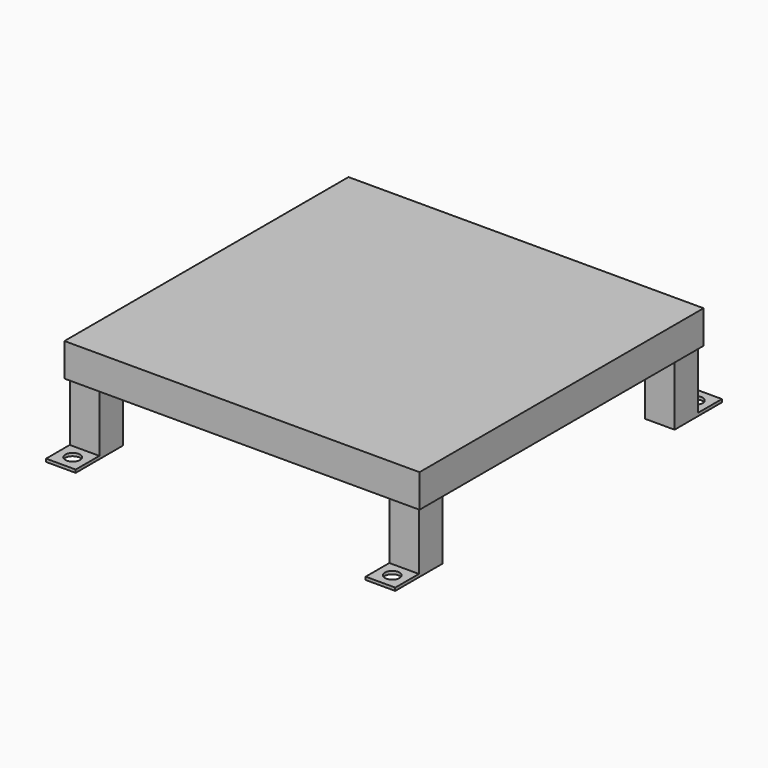
from build123d import *

# Parameters (mm, degrees)
F0_W         = 304.8
F0_H         = 304.8
F1_DEPTH     = 3
F2_W         = 304.8
F2_H         = 304.8
F3_DEPTH     = 25.4
F4_T         = -2.54
F5_W         = 25.4
F5_H         = 25.4
F6_DEPTH     = 76.2
F7_T         = 2.54
F7_T3_DEPTH  = 30.48
F7_T5_DEPTH  = 30.48
F7_T7_DEPTH  = 30.94
F7_T9_DEPTH  = 304.8
F7_T11_DEPTH = 279.4
F7_T13_DEPTH = 279.4
F7_T15_DEPTH = 304.8
F8_W         = 25.4
F8_H         = 25.4
F8_W_2       = 20.32
F8_H_2       = 20.32
F9_DEPTH     = 76.2
F10_W        = 25.4
F10_H        = 50.8
F10_R        = 6.3459053742
F11_DEPTH    = 2.54
F12_W        = 25.4
F12_H        = 50.8
F12_R        = 6.35
F13_DEPTH    = 2.54
F14_W        = 25.4
F14_H        = 50.8
F14_R        = 6.35
F15_DEPTH    = 2.54
F16_W        = 25.4
F16_H        = 50.8
F16_R        = 6.35
F17_DEPTH    = 2.54


# Not quite as in the source:
# - a shell that OpenCascade refuses in one call is made with other operations: the cavity is built on its own and cut out


with BuildPart() as f1:
    # F0 (on Top) → F1 (new body)
    with BuildSketch(Plane.XY):
        with Locations((152.4, -152.4)):
            Rectangle(F0_W, F0_H)
    extrude(amount=F1_DEPTH)

    # F2 (on face) → F3 (join)
    with BuildSketch(Plane(origin=(0, 0, 0), x_dir=(1, 0, 0), z_dir=(0, 0, -1))):
        with Locations((152.4, 152.4)):
            Rectangle(F2_W, F2_H)
    extrude(amount=F3_DEPTH)

    # F4
    f4_openings = [f1.faces().sort_by_distance(p)[0] for p in [
        (152.4, -152.4, -25.4),
    ]]
    offset(amount=F4_T, openings=f4_openings)

    # F5 (on face) → F6 (join)
    with BuildSketch(Plane(origin=(0, 0, 0.46), x_dir=(1, 0, 0), z_dir=(0, 0, -1))):
        with Locations((289.56, 289.56)):
            Rectangle(F5_W, F5_H)
    extrude(amount=F6_DEPTH)

    # F7: shell of thickness 2.54, made by hand


with BuildPart() as f7_core1:
    # F7_t2: copy of F1
    add(f1.part)

    # the walls: a layer under each face that stays
    f7_faces = [f7_core1.faces().sort_by_distance(p)[0] for p in [
        (152.4, -304.8, -11.2),
        (152.4, -152.4, 3),
        (304.8, -152.4, -11.2),
        (2.38125, -120.4148148148, -25.4),
        (0, -152.4, -11.2),
        (152.4, 0, -11.2),
        (2.54, -152.4, -12.47),
        (289.56, -302.26, -50.57),
        (139.7, -302.26, -12.47),
        (302.26, -139.7, -12.47),
        (302.26, -289.56, -50.57),
        (152.4, -2.54, -12.47),
        (152.4, -152.4, 0.46),
        (276.86, -289.56, -37.64),
        (289.56, -276.86, -37.64),
    ]]
    thicken(f7_faces, amount=-F7_T, mode=Mode.SUBTRACT)

    # F7_s4 → F7_t3 (cut)
    with BuildSketch(Plane.YZ.offset(274.32)):
        Polygon((-302.2854, -25.4254), (-302.26, -22.86), (-299.72, -22.86), (-299.72, -25.4), align=None)
        Polygon((-276.8346, 0.4346), (-276.86, 3), (-279.4, 3), (-279.4, 0.46), align=None)
    extrude(amount=F7_T3_DEPTH, mode=Mode.SUBTRACT)

    # F7_s6 → F7_t5 (cut)
    with BuildSketch(Plane.XZ.offset(274.32)):
        Polygon((302.2854, -25.4254), (302.26, -22.86), (299.72, -22.86), (299.72, -25.4), align=None)
        Polygon((276.8346, 0.4346), (276.86, 3), (279.4, 3), (279.4, 0.46), align=None)
    extrude(amount=F7_T5_DEPTH, mode=Mode.SUBTRACT)

    # F7_s8 → F7_t7 (cut)
    with BuildSketch(Plane.XY.offset(-27.94)):
        Polygon((2.5654, -2.5654), (0, -2.54), (0, 0), (2.54, 0), align=None)
        Polygon((2.5654, -302.2346), (0, -302.26), (0, -304.8), (2.54, -304.8), align=None)
        Polygon((276.8346, -302.2346), (276.86, -304.8), (279.4, -304.8), (279.4, -302.26), align=None)
        Polygon((302.2346, -2.5654), (304.8, -2.54), (304.8, 0), (302.26, 0), align=None)
        Polygon((302.2346, -276.8346), (304.8, -276.86), (304.8, -279.4), (302.26, -279.4), align=None)
    extrude(amount=F7_T7_DEPTH, mode=Mode.SUBTRACT)

    # F7_s10 → F7_t9 (cut)
    with BuildSketch(Plane.XZ):
        Polygon((2.5654, 0.4346), (0, 0.46), (0, 3), (2.54, 3), align=None)
    extrude(amount=F7_T9_DEPTH, mode=Mode.SUBTRACT)

    # F7_s12 → F7_t11 (cut)
    with BuildSketch(Plane.YZ):
        Polygon((-302.2346, 0.4346), (-304.8, 0.46), (-304.8, 3), (-302.26, 3), align=None)
    extrude(amount=F7_T11_DEPTH, mode=Mode.SUBTRACT)

    # F7_s14 → F7_t13 (cut)
    with BuildSketch(Plane.XZ):
        Polygon((302.2346, 0.4346), (304.8, 0.46), (304.8, 3), (302.26, 3), align=None)
    extrude(amount=F7_T13_DEPTH, mode=Mode.SUBTRACT)

    # F7_s16 → F7_t15 (cut)
    with BuildSketch(Plane.YZ):
        Polygon((-2.5654, 0.4346), (0, 0.46), (0, 3), (-2.54, 3), align=None)
    extrude(amount=F7_T15_DEPTH, mode=Mode.SUBTRACT)


with BuildPart() as f1_1:
    add(f1.part)

    # what is left inside the walls is the cavity
    f7_cavity = [f7_core1.part.solids().sort_by_distance(p)[0] for p in [
        (290.83, -279.4254, -50.34),
    ]]
    add(f7_cavity, mode=Mode.SUBTRACT)

    # F8 (on face) → F9 (join)
    with BuildSketch(Plane(origin=(0, 0, 0.46), x_dir=(1, 0, 0), z_dir=(0, 0, -1))):
        with Locations((15.24, 15.24)):
            Rectangle(F8_W, F8_H)
        with Locations((15.24, 15.24)):
            Rectangle(F8_W_2, F8_H_2, mode=Mode.SUBTRACT)
        with Locations((289.56, 15.24)):
            Rectangle(F8_W, F8_H)
        Polygon((279.4, 5.08), (279.4, 15.24), (279.4, 25.4), (299.72, 25.4), (299.72, 5.08), align=None, mode=Mode.SUBTRACT)
        with Locations((15.24, 289.56)):
            Rectangle(F8_W, F8_H)
        Polygon((25.4, 279.4), (15.24, 279.4), (5.08, 279.4), (5.08, 299.72), (25.4, 299.72), align=None, mode=Mode.SUBTRACT)
    extrude(amount=F9_DEPTH)

    # F10 (on face) → F11 (join)
    with BuildSketch(Plane(origin=(0, 0, -75.74), x_dir=(1, 0, 0), z_dir=(0, 0, -1))):
        with Locations((289.56, 2.54)):
            Rectangle(F10_W, F10_H)
        with Locations((289.56, -10.1621253416)):
            Circle(F10_R, mode=Mode.SUBTRACT)
    extrude(amount=F11_DEPTH)

    # F12 (on face) → F13 (join)
    with BuildSketch(Plane(origin=(0, 0, -75.74), x_dir=(1, 0, 0), z_dir=(0, 0, -1))):
        with Locations((15.24, 2.54)):
            Rectangle(F12_W, F12_H)
        with Locations((15.24, -10.16)):
            Circle(F12_R, mode=Mode.SUBTRACT)
    extrude(amount=F13_DEPTH)

    # F14 (on face) → F15 (join)
    with BuildSketch(Plane(origin=(0, 0, -75.74), x_dir=(1, 0, 0), z_dir=(0, 0, -1))):
        with Locations((15.24, 302.26)):
            Rectangle(F14_W, F14_H)
        with Locations((15.24, 314.96)):
            Circle(F14_R, mode=Mode.SUBTRACT)
    extrude(amount=F15_DEPTH)

    # F16 (on face) → F17 (join)
    with BuildSketch(Plane(origin=(0, 0, -75.74), x_dir=(1, 0, 0), z_dir=(0, 0, -1))):
        with Locations((289.56, 302.26)):
            Rectangle(F16_W, F16_H)
        with Locations((289.56, 314.96)):
            Circle(F16_R, mode=Mode.SUBTRACT)
    extrude(amount=F17_DEPTH)


solid = f1_1.part
